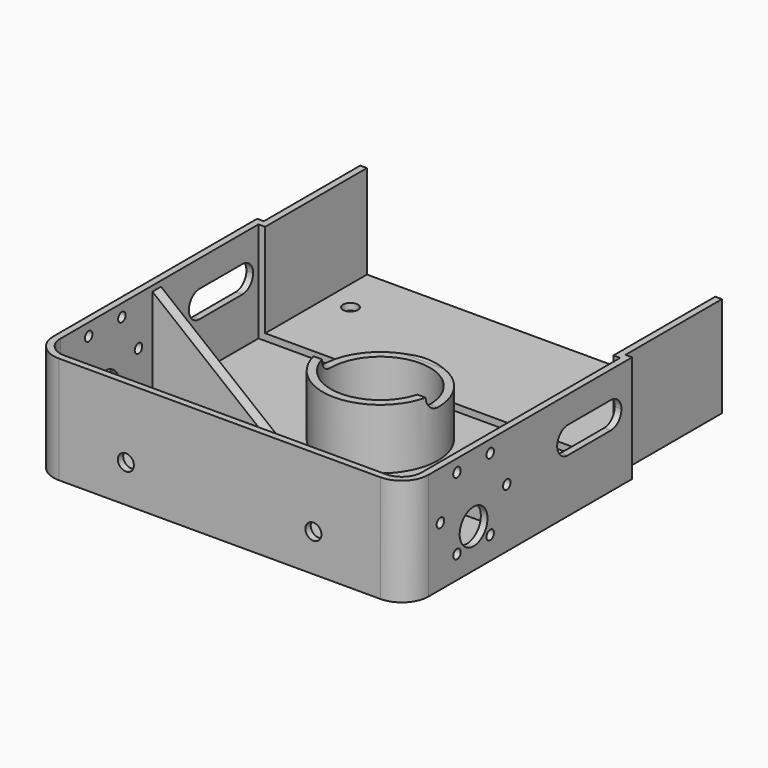
from build123d import *

# Parameters (mm, degrees)
F0_W             = 140
F0_H             = 150
F1_DEPTH         = 40
F2_R             = 10
F3_W             = 200
F3_H             = 100
F4_DEPTH         = 2.5
F5_W             = 40
F5_H             = 60
F6_DEPTH         = 200
F7_T             = 2.5
F7_T3_DEPTH      = 42.5
F7_T5_DEPTH      = 140
F8_R             = 6
F9_DEPTH         = 25
F10_R            = 21.5
F10_R_2          = 18.5
F11_DEPTH        = 25
F12_R            = 2.75
F13_DEPTH        = 25
F14_R            = 6.5
F15_DEPTH        = 300
F15_DEPTH_BACK   = 300
F16_R            = 3
F17_DEPTH        = 200
F18_R            = 1.75
F19_DEPTH        = 200
F19_COPIES_COUNT = 6
F20_R            = 1.75
F21_DEPTH        = 12.5
F21_COPIES_COUNT = 4
F23_START        = -28
F23_DEPTH        = 4
F25_DEPTH        = 150
F26_R            = 3.5
F27_DEPTH        = 25


# Not quite as in the source:
# - a pattern or mirror of a feature is missing from the dataset's text; its kind, count and spacing are read off the source's solid
# - a shell that OpenCascade refuses in one call is made with other operations: the cavity is built on its own and cut out


with BuildPart() as f1:
    # F0 (on Top) → F1 (new body)
    with BuildSketch(Plane.XY):
        with Locations((0, 50)):
            Rectangle(F0_W, F0_H)
    extrude(amount=F1_DEPTH)

    # F2
    f2_edges = [f1.edges().sort_by_distance(p)[0] for p in [
        (-70, -25, 20),
        (70, -25, 20),
    ]]
    fillet(f2_edges, radius=F2_R)

    # F3 (on Top) → F4 (cut)
    with BuildSketch(Plane.XY):
        with Locations((0, 130)):
            Rectangle(F3_W, F3_H)
    extrude(amount=F4_DEPTH, mode=Mode.SUBTRACT)

    # F5 (on Top) → F6 (cut)
    with BuildSketch(Plane.XY):
        with Locations((-87.5, 110)):
            Rectangle(F5_W, F5_H)
        with Locations((87.5, 110)):
            Rectangle(F5_W, F5_H)
    extrude(amount=F6_DEPTH, mode=Mode.SUBTRACT)

    # F7: shell of thickness 2.5, made by hand


with BuildPart() as f7_core1:
    # F7_t2: copy of F1
    add(f1.part)

    # the walls: a layer under each face that stays
    f7_faces = [f7_core1.faces().sort_by_distance(p)[0] for p in [
        (-70, 32.5, 20),
        (-67.0710678119, -22.0710678119, 20),
        (0, -25, 20),
        (67.0710678119, -22.0710678119, 20),
        (70, 32.5, 20),
        (67.5, 102.5, 21.25),
        (0, 102.5, 2.5),
        (-67.5, 102.5, 21.25),
        (-65.3333333333, 80, 1.3333333333),
        (0, 27.5, 0),
    ]]
    thicken(f7_faces, amount=-F7_T, mode=Mode.SUBTRACT)

    # F7_s4 → F7_t3 (cut)
    with BuildSketch(Plane.XY):
        Polygon((67.525, 80.025), (65, 80), (65, 77.5), (67.5, 77.5), align=None)
        Polygon((-67.525, 80.025), (-65, 80), (-65, 77.5), (-67.5, 77.5), align=None)
    extrude(amount=F7_T3_DEPTH, mode=Mode.SUBTRACT)

    # F7_s6 → F7_t5 (cut)
    with BuildSketch(Plane.YZ.offset(-70)):
        Polygon((80.025, 2.475), (80, 5), (77.5, 5), (77.5, 2.5), align=None)
    extrude(amount=F7_T5_DEPTH, mode=Mode.SUBTRACT)


with BuildPart() as f1_1:
    add(f1.part)

    # what is left inside the walls is the cavity
    f7_cavity = [f7_core1.part.solids().sort_by_distance(p)[0] for p in [
        (0, 26.666667, 39.975),
    ]]
    add(f7_cavity, mode=Mode.SUBTRACT)

    # F8 (on Top) → F9 (cut)
    with BuildSketch(Plane.XY):
        with Locations((0, 50)):
            Circle(F8_R)
    extrude(amount=F9_DEPTH, mode=Mode.SUBTRACT)

    # F10 (on Top) → F11 (join)
    with BuildSketch(Plane.XY):
        with Locations((0, 50)):
            Circle(F10_R)
        with Locations((0, 50)):
            Circle(F10_R_2, mode=Mode.SUBTRACT)
    extrude(amount=F11_DEPTH)

    # F12 (on Top) → F13 (cut)
    with BuildSketch(Plane.XY):
        with Locations((-55.8614357137, -5.8614357137)):
            Circle(F12_R)
        with Locations((55.8614357137, -5.8614357137)):
            Circle(F12_R)
        with Locations((55.8614357137, 105.8614357137)):
            Circle(F12_R)
        with BuildLine():
            ThreePointArc((-53.9168920655, 103.9168920655), (-53.3207669993, 104.8090562747), (-53.1114357137, 105.8614357137))
            ThreePointArc((-53.1114357137, 105.8614357137), (-58.4021044281, 106.9138151527), (-53.9168920655, 103.9168920655))
        make_face()
    extrude(amount=F13_DEPTH, mode=Mode.SUBTRACT)

    # F14 (on Right) → F15 (cut, two sides)
    with BuildSketch(Plane.YZ) as f15_sk:
        with Locations((6, 14.5)):
            Circle(F14_R)
    extrude(amount=-F15_DEPTH, mode=Mode.SUBTRACT)
    extrude(f15_sk.sketch, amount=F15_DEPTH_BACK, mode=Mode.SUBTRACT)

    # F16 (on Front) → F17 (cut)
    with BuildSketch(Plane.XZ):
        with Locations((-35, 14)):
            Circle(F16_R)
        with Locations((35, 14)):
            Circle(F16_R)
    extrude(amount=F17_DEPTH, mode=Mode.SUBTRACT)

    # F18 (on Right) → F19 (cut, symmetric)
    with BuildSketch(Plane.YZ):
        with Locations((-1.75, 8.5766062413)):
            Circle(F18_R)
    f19 = extrude(amount=F19_DEPTH, both=True, mode=Mode.SUBTRACT)

    # F19_copies: F19 ×6 about axis
    f19_copies_axis = Axis((0, 6, 22), (1, 0, 0))
    for i in range(1, F19_COPIES_COUNT):
        add(f19.rotate(f19_copies_axis, i * 360 / F19_COPIES_COUNT), mode=Mode.SUBTRACT)

    # F20 (on Top) → F21 (cut, symmetric)
    with BuildSketch(Plane.XY):
        with Locations((0, 37.5)):
            Circle(F20_R)
    f21 = extrude(amount=F21_DEPTH, both=True, mode=Mode.SUBTRACT)

    # F21_copies: F21 ×4 about axis
    f21_copies_axis = Axis((0, 50, 0), (0, 0, 1))
    for i in range(1, F21_COPIES_COUNT):
        add(f21.rotate(f21_copies_axis, i * 360 / F21_COPIES_COUNT), mode=Mode.SUBTRACT)

    # F22 (on Front) → F23 (join)
    with BuildSketch(Plane.XZ.offset(F23_START)):
        Polygon((-70, 40), (-70, 0), (-20, 0), align=None)
        Polygon((70, 40), (20, 0), (70, 0), align=None)
    extrude(amount=-F23_DEPTH)

    # F24 (on Right) → F25 (cut, symmetric)
    with BuildSketch(Plane.YZ):
        with BuildLine():
            Line((50, 20), (50, 30))
            ThreePointArc((50, 30), (45, 25), (50, 20))
        make_face()
        with BuildLine():
            ThreePointArc((55, 25), (53.5355339059, 28.5355339059), (50, 30))
            Line((50, 30), (50, 20))
            ThreePointArc((50, 20), (53.5355339059, 21.4644660941), (55, 25))
        make_face()
        with BuildLine():
            Line((70, 30), (50, 30))
            ThreePointArc((50, 30), (53.5355339059, 28.5355339059), (55, 25))
            ThreePointArc((55, 25), (53.5355339059, 21.4644660941), (50, 20))
            Line((50, 20), (70, 20))
            ThreePointArc((70, 20), (65, 25), (70, 30))
        make_face()
        with BuildLine():
            Line((70, 20), (70, 30))
            ThreePointArc((70, 30), (65, 25), (70, 20))
        make_face()
        with BuildLine():
            ThreePointArc((75, 25), (73.5355339059, 28.5355339059), (70, 30))
            Line((70, 30), (70, 20))
            ThreePointArc((70, 20), (73.5355339059, 21.4644660941), (75, 25))
        make_face()
    extrude(amount=F25_DEPTH, both=True, mode=Mode.SUBTRACT)

    # F26 (on Top) → F27 (cut)
    with BuildSketch(Plane.XY):
        with Locations((0, -15)):
            Circle(F26_R)
    extrude(amount=F27_DEPTH, mode=Mode.SUBTRACT)


solid = f1_1.part
